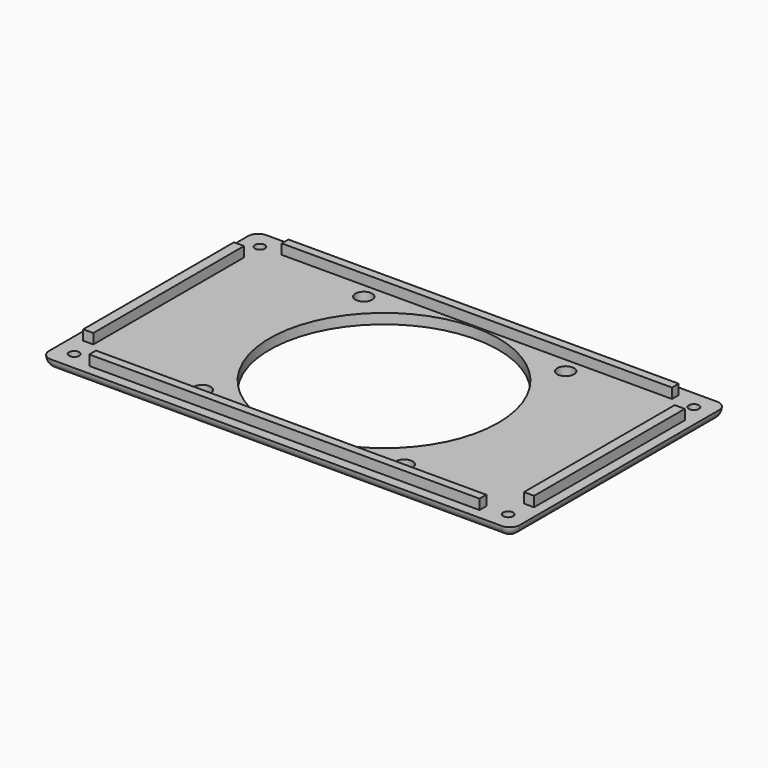
from build123d import *

# Parameters (mm, degrees)
F0_W     = 116
F0_H     = 2.5
F1_DEPTH = 6
F0_W_2   = 3
F0_H_2   = 56
F0_W_3   = 140
F0_H_3   = 80
F0_R     = 1.5
F0_R_2   = 2.5
F0_R_3   = 34
F2_DEPTH = 3
F3_R     = 2.99999


# Not quite as in the source:
# - a fillet or chamfer is up to 0.001 mm smaller than in the source, because OpenCascade refuses the exact size


with BuildPart() as f1:
    # F0 (on Top) → F1 (new body)
    with BuildSketch(Plane.XY):
        with Locations((70, 75.75)):
            Rectangle(F0_W, F0_H)
    extrude(amount=F1_DEPTH)



with BuildPart() as f1b:
    # F0 (on Top) → F1, piece 2 (new body)
    with BuildSketch(Plane.XY):
        with Locations((70, 4.25)):
            Rectangle(F0_W, F0_H)
    extrude(amount=F1_DEPTH)


with BuildPart() as f1c:
    # F0 (on Top) → F1, piece 3 (new body)
    with BuildSketch(Plane.XY):
        with Locations((4.5, 40)):
            Rectangle(F0_W_2, F0_H_2)
    extrude(amount=F1_DEPTH)


with BuildPart() as f1d:
    # F0 (on Top) → F1, piece 4 (new body)
    with BuildSketch(Plane.XY):
        with Locations((135.5, 40)):
            Rectangle(F0_W_2, F0_H_2)
    extrude(amount=F1_DEPTH)


with BuildPart() as f1_1:
    add(f1.part)

    add(f1b.part)  # F2 merges F1b

    add(f1c.part)  # F2 merges F1c

    add(f1d.part)  # F2 merges F1d
    # F0 (on Top) → F2 (join)
    with BuildSketch(Plane.XY):
        with Locations((70, 40)):
            Rectangle(F0_W_3, F0_H_3)
        with Locations((5.5, 5.5)):
            Circle(F0_R, mode=Mode.SUBTRACT)
        with Locations((40, 10)):
            Circle(F0_R_2, mode=Mode.SUBTRACT)
        with Locations((70, 4.25)):
            Rectangle(F0_W, F0_H, mode=Mode.SUBTRACT)
        with Locations((100, 10)):
            Circle(F0_R_2, mode=Mode.SUBTRACT)
        with Locations((134.5, 5.5)):
            Circle(F0_R, mode=Mode.SUBTRACT)
        with Locations((4.5, 40)):
            Rectangle(F0_W_2, F0_H_2, mode=Mode.SUBTRACT)
        with Locations((5.5, 74.5)):
            Circle(F0_R, mode=Mode.SUBTRACT)
        with Locations((40, 70)):
            Circle(F0_R_2, mode=Mode.SUBTRACT)
        with Locations((70, 40)):
            Circle(F0_R_3, mode=Mode.SUBTRACT)
        with Locations((135.5, 40)):
            Rectangle(F0_W_2, F0_H_2, mode=Mode.SUBTRACT)
        with Locations((70, 75.75)):
            Rectangle(F0_W, F0_H, mode=Mode.SUBTRACT)
        with Locations((100, 70)):
            Circle(F0_R_2, mode=Mode.SUBTRACT)
        with Locations((134.5, 74.5)):
            Circle(F0_R, mode=Mode.SUBTRACT)
    extrude(amount=F2_DEPTH)

    # F3 (radius 3 in the source; OpenCascade refuses exactly that, so slightly less here)
    f3_edges = [f1_1.edges().sort_by_distance(p)[0] for p in [
        (140, 40, 0),
        (140, 80, 1.5),
        (0, 0, 1.5),
        (0, 80, 1.5),
        (140, 0, 1.5),
        (70, 0, 0),
        (70, 80, 0),
        (0, 40, 0),
    ]]
    fillet(f3_edges, radius=F3_R)


solid = f1_1.part
